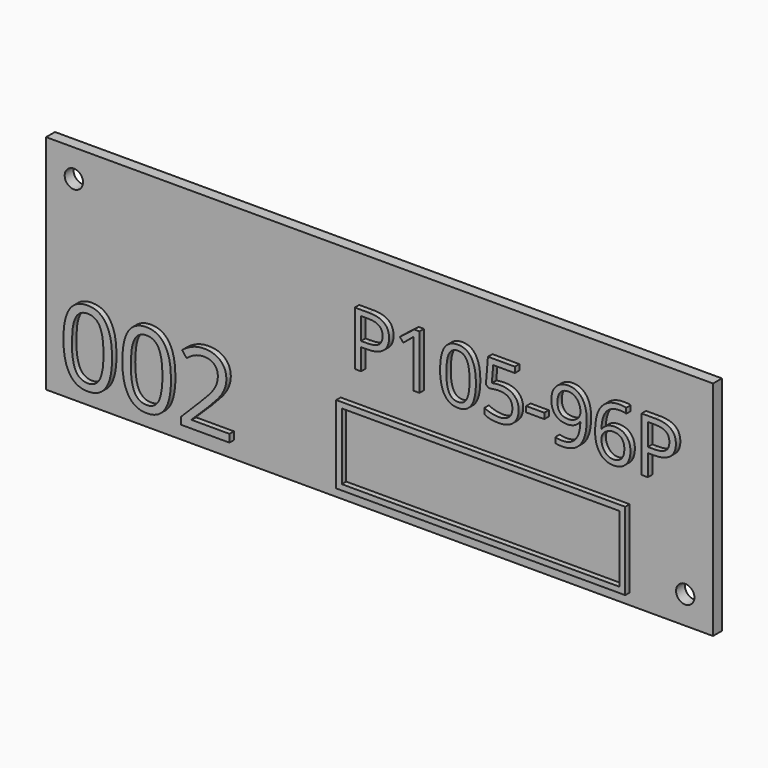
from build123d import *

# Parameters (mm, degrees)
F0_W         = 120
F0_H         = 40
F1_DEPTH     = 2
F3_D         = 3.3
F4_TEXT_SIZE = 13.6426617401
F5_DEPTH     = 1
F6_TEXT_SIZE = 18.5356140827
F7_DEPTH     = 1
F8_W         = 52
F8_H         = 14
F8_W_2       = 49.99999962
F8_H_2       = 11.99999962
F9_DEPTH     = 1


# Not quite as in the source:
# - Text() gives the source's letters only with a copy of the font that has no kerning and outlines rounded to 1/6400 em; it was checked with that copy


with BuildPart() as f1:
    # F0 (on Front) → F1 (new body)
    with BuildSketch(Plane.XZ):
        Rectangle(F0_W, F0_H)
    extrude(amount=F1_DEPTH)

    # F3 (through all)
    with Locations(Plane.XZ.offset(2)):
        with Locations((-55, 15), (55, -15)):
            Hole(F3_D / 2)

    # F4 (on face) → F5 (join)
    with BuildSketch(Plane.XZ.offset(2)):
        with Locations((-5, 2)):
            Text('P105-96P', F4_TEXT_SIZE, font='Open Sans', text_align=(TextAlign.LEFT, TextAlign.BOTTOM))
    extrude(amount=F5_DEPTH)

    # F6 (on face) → F7 (join)
    with BuildSketch(Plane.XZ.offset(2)):
        with Locations((-57, -17)):
            Text('002', F6_TEXT_SIZE, font='Open Sans', text_align=(TextAlign.LEFT, TextAlign.BOTTOM))
    extrude(amount=F7_DEPTH)

    # F8 (on face) → F9 (join)
    with BuildSketch(Plane.XZ.offset(2)):
        with Locations((19, -11)):
            Rectangle(F8_W, F8_H)
        with Locations((19, -11)):
            Rectangle(F8_W_2, F8_H_2, mode=Mode.SUBTRACT)
    extrude(amount=F9_DEPTH)


solid = f1.part
